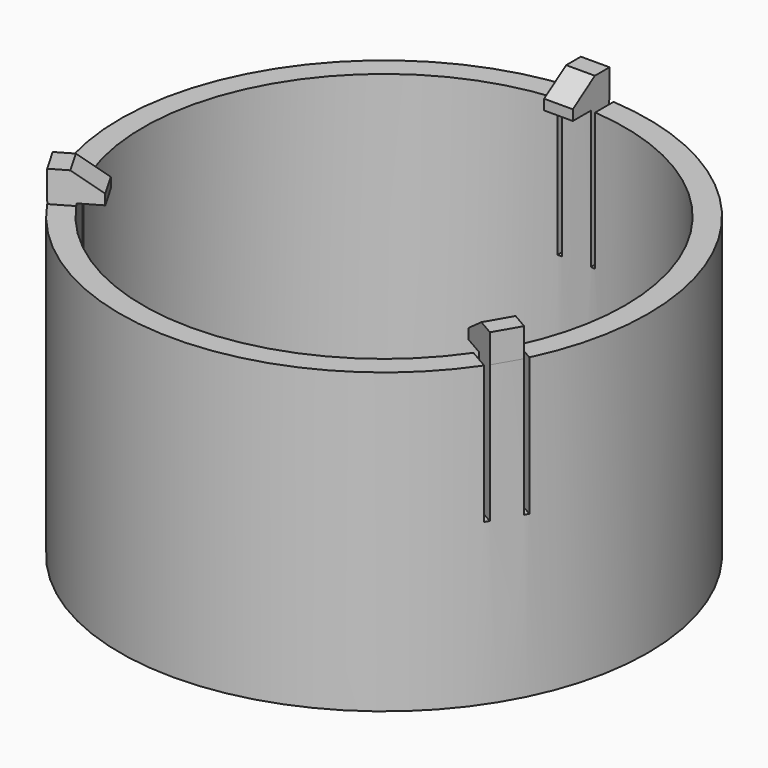
from build123d import *

# Parameters (mm, degrees)
F0_R            = 29.21
F1_DEPTH        = 33.02
F2_R            = 26.67
F3_DEPTH        = 30.48
F4_W            = 3.175
F4_H            = 5.08
F5_DEPTH        = 3.175
F5_COPIES_COUNT = 3
F7_DEPTH        = 3.175
F7_COPIES_COUNT = 3
F8_W            = 0.508
F8_H            = 15.24
F9_DEPTH        = 5.08
F9_COPIES_COUNT = 3


# Not quite as in the source:
# - a pattern or mirror of a feature is missing from the dataset's text; its kind, count and spacing are read off the source's solid


with BuildPart() as f1:
    # F0 (on Top) → F1 (new body)
    with BuildSketch(Plane.XY):
        Circle(F0_R)
    extrude(amount=F1_DEPTH)

    # F2 (on face) → F3 (cut)
    with BuildSketch(Plane.XY.offset(33.02)):
        Circle(F2_R)
    extrude(amount=-F3_DEPTH, mode=Mode.SUBTRACT)

    # F4 (on face) → F5 (join)
    with BuildSketch(Plane.XY.offset(33.02)):
        with Locations((0, 26.67)):
            Rectangle(F4_W, F4_H)
    f5 = extrude(amount=F5_DEPTH)

    # F5_copies: F5 ×3 about axis
    f5_copies_axis = Axis((0, 0, 0), (0, 0, 1))
    for i in range(1, F5_COPIES_COUNT):
        add(f5.rotate(f5_copies_axis, i * 360 / F5_COPIES_COUNT))

    # F6 (on face) → F7 (cut, through all)
    with BuildSketch(Plane(origin=(-1.5875, 0, 0), x_dir=(0, -1, 0), z_dir=(-1, 0, 0))):
        Polygon((-24.13, 36.195), (-27.178, 36.195), (-24.13, 34.163), align=None)
    f7 = extrude(amount=-F7_DEPTH, mode=Mode.SUBTRACT)

    # F7_copies: F7 ×3 about axis
    f7_copies_axis = Axis((0, 0, 0), (0, 0, 1))
    for i in range(1, F7_COPIES_COUNT):
        add(f7.rotate(f7_copies_axis, i * 360 / F7_COPIES_COUNT), mode=Mode.SUBTRACT)

    # F8 (on face) → F9 (cut)
    with BuildSketch(Plane(origin=(0, 29.21, 0), x_dir=(-1, 0, 0), z_dir=(0, 1, 0))):
        with Locations((1.8415, 25.4)):
            Rectangle(F8_W, F8_H)
        with Locations((-1.8415, 25.4)):
            Rectangle(F8_W, F8_H)
    f9 = extrude(amount=-F9_DEPTH, mode=Mode.SUBTRACT)

    # F9_copies: F9 ×3 about axis
    f9_copies_axis = Axis((0, 0, 0), (0, 0, 1))
    for i in range(1, F9_COPIES_COUNT):
        add(f9.rotate(f9_copies_axis, i * 360 / F9_COPIES_COUNT), mode=Mode.SUBTRACT)


solid = f1.part
